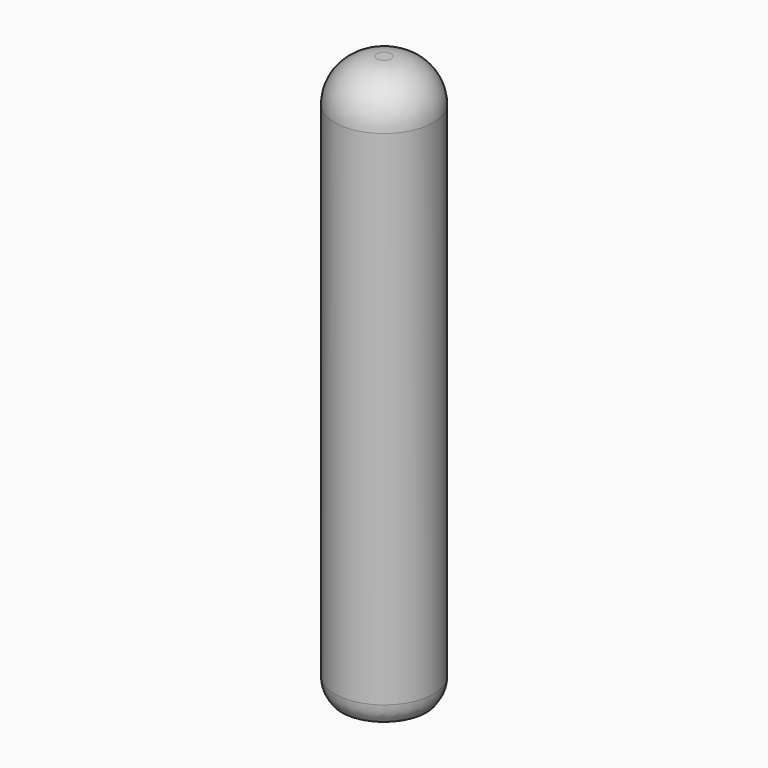
from build123d import *

# Parameters (mm, degrees)
F0_R     = 7
F1_DEPTH = 80
F2_R     = 6
F3_T     = -1


# Not quite as in the source:
# - a fillet or chamfer that OpenCascade refuses, or shapes differently, is made with other operations: its cross-section is extruded or revolved along the edge and cut away or added


with BuildPart() as f1:
    # F0 (on Top) → F1 (new body)
    with BuildSketch(Plane.XY):
        Circle(F0_R)
    extrude(amount=F1_DEPTH)

    # F2
    f2_edges = [f1.edges().sort_by_distance(p)[0] for p in [
        (-7, 0, 80),
    ]]
    fillet(f2_edges, radius=F2_R)

    # F3
    f3_openings = [f1.faces().sort_by_distance(p)[0] for p in [
        (0, 0, 0),
    ]]
    offset(amount=F3_T, openings=f3_openings)

    # F4: fillet of radius 4 on 1 edges, made by hand

    # F4_s1 → F4_t2 (revolve, cut)
    with BuildSketch(Plane.XZ):
        with BuildLine():
            ThreePointArc((7, 2.6457513111), (6.7416573868, 1.2315377487), (6, 0))
            Line((6, 0), (7, 0))
            Line((7, 0), (7, 2.6457513111))
        make_face()
    revolve(axis=Axis((0, 0, 0), (0, 0, 1)), mode=Mode.SUBTRACT)


solid = f1.part
